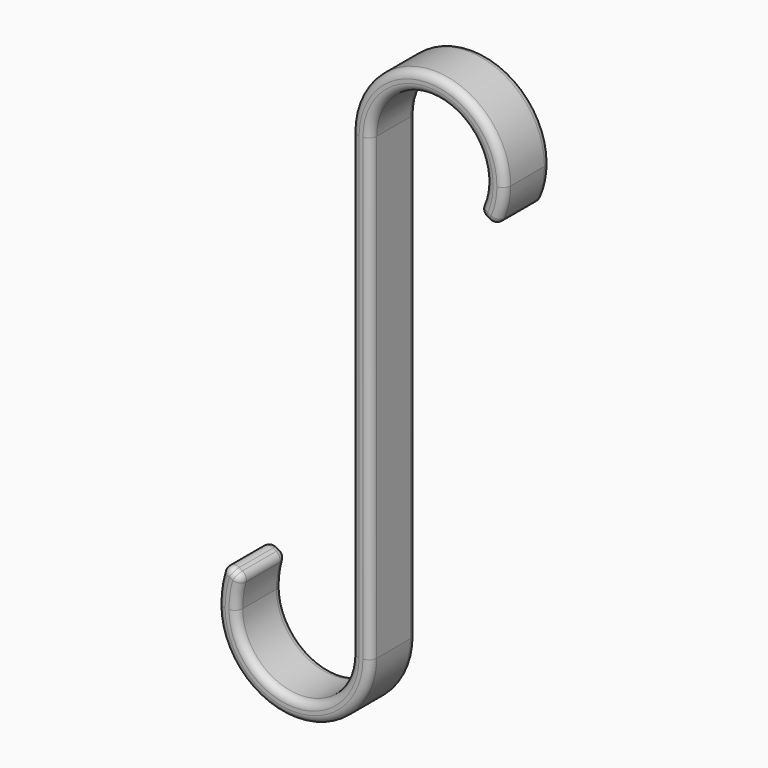
from build123d import *

# Parameters (mm, degrees)
F1_DEPTH = 19.05
F2_R     = 2.54


# Not quite as in the source:
# - a feature names something its author has since deleted; it is built from what else it names


with BuildPart() as f1:
    # F0 (on Front) → F1 (new body)
    with BuildSketch(Plane.XZ):
        with BuildLine():
            ThreePointArc((13.97, 0), (-11.43, 25.4), (-36.83, 0))
            Line((-36.83, 0), (-36.83, -152.4))
            ThreePointArc((-36.83, -152.4), (-55.88, -171.45), (-74.93, -152.4))
            ThreePointArc((-74.93, -152.4), (-74.5044281022, -147.3179462529), (-73.2395664242, -142.377449652))
            Line((-73.2395664242, -142.377449652), (-78.7388277382, -139.202449652))
            ThreePointArc((-78.7388277382, -139.202449652), (-80.638925247, -145.6800131761), (-81.28, -152.4))
            ThreePointArc((-81.28, -152.4), (-55.88, -177.8), (-30.48, -152.4))
            Line((-30.48, -152.4), (-30.48, 0))
            ThreePointArc((-30.48, 0), (-6.4994971908, 18.4008869908), (5.0677839421, -9.525))
            Line((5.0677839421, -9.525), (10.5670452561, -12.7))
            ThreePointArc((10.5670452561, -12.7), (13.1045159877, -6.5740037456), (13.97, 0))
        make_face()
    extrude(amount=F1_DEPTH)

    # F2
    f2_edges = [f1.edges().sort_by_distance(p)[0] for p in [
        (-73.239566, -9.525, -142.37745),
        (-78.738828, -9.525, -139.20245),
        (-75.989197, 0, -140.78995),
        (-75.989197, -19.05, -140.78995),
        (5.067784, -9.525, -9.525),
        (10.567045, -9.525, -12.7),
        (7.817415, 0, -11.1125),
        (7.817415, -19.05, -11.1125),
        (-55.88, 0, -177.8),
        (-30.48, 0, -76.2),
        (-6.499497, 0, 18.400887),
        (-4.855996, 0, 24.534516),
        (-36.83, 0, -76.2),
        (-55.88, 0, -171.45),
        (-74.504428, 0, -147.317946),
        (-80.638925, 0, -145.680013),
        (-55.88, -19.05, -177.8),
        (-30.48, -19.05, -76.2),
        (-6.499497, -19.05, 18.400887),
        (-4.855996, -19.05, 24.534516),
        (-36.83, -19.05, -76.2),
        (-55.88, -19.05, -171.45),
        (-74.504428, -19.05, -147.317946),
        (-80.638925, -19.05, -145.680013),
    ]]
    fillet(f2_edges, radius=F2_R)


solid = f1.part
